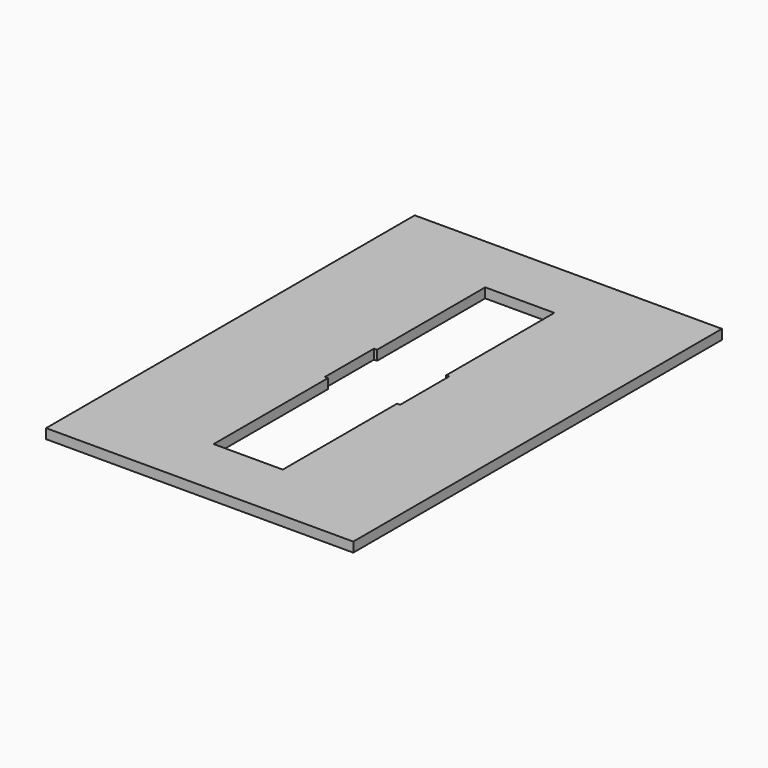
from build123d import *

# Parameters (mm, degrees)
F0_W     = 200
F0_H     = 300
F1_DEPTH = 6.35
F2_W     = 2
F2_H     = 40
F3_DEPTH = 25.4


# Not quite as in the source:
# - a length typed as a fraction of an inch, garbled in the dataset ("3 / 203.2 mm" for 3/8 in), is restored


with BuildPart() as f1:
    # F0 (on Top) → F1 (new body)
    with BuildSketch(Plane.XY):
        Rectangle(F0_W, F0_H)
    extrude(amount=F1_DEPTH)

    # F2 (on face) → F3 (cut)
    with BuildSketch(Plane.XY.offset(6.35)):
        Polygon((22.5, 22.48), (22.5, 110.5), (-22.5, 110.5), (-22.5, 22.48), (-22.5, -17.52), (-22.5, -110.5), (22.5, -110.5), (22.5, -17.52), align=None)
        with Locations((23.5, 2.48)):
            Rectangle(F2_W, F2_H)
        with Locations((-23.5, 2.48)):
            Rectangle(F2_W, F2_H)
    extrude(amount=-F3_DEPTH, mode=Mode.SUBTRACT)


solid = f1.part
